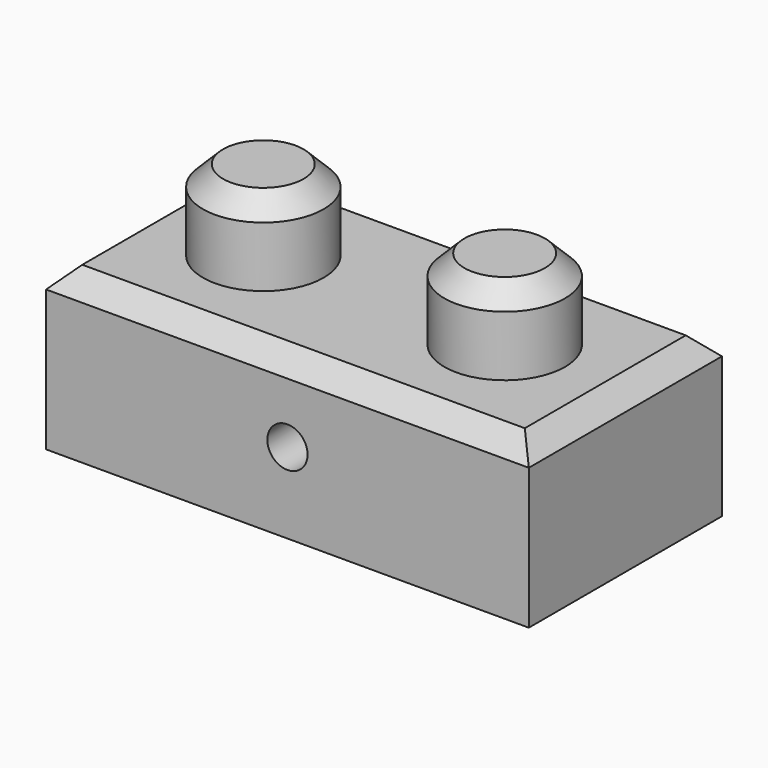
from build123d import *

# Parameters (mm, degrees)
F0_W     = 76.2
F0_H     = 38.1
F1_DEPTH = 25.4
F2_R     = 9.525
F3_DEPTH = 12.7
F4_SIZE2 = 3.175
F4_SIZE  = 3.175
F5_T     = 7.9375
F6_R     = 3.175
F7_DEPTH = 38.1


# Not quite as in the source:
# - a shell that OpenCascade refuses in one call is made with other operations: the cavity is built on its own and cut out


with BuildPart() as f1:
    # F0 (on Top) → F1 (new body)
    with BuildSketch(Plane.XY):
        with Locations((38.1, -19.05)):
            Rectangle(F0_W, F0_H)
    extrude(amount=F1_DEPTH)

    # F2 (on face) → F3 (join)
    with BuildSketch(Plane.XY.offset(25.4)):
        with Locations((19.05, -19.05)):
            Circle(F2_R)
        with Locations((57.15, -19.05)):
            Circle(F2_R)
    extrude(amount=F3_DEPTH)

    # F4
    f4_edges = [f1.edges().sort_by_distance(p)[0] for p in [
        (9.525, -19.05, 38.1),
        (47.625, -19.05, 38.1),
        (38.1, -38.1, 25.4),
        (76.2, -19.05, 25.4),
        (38.1, 0, 25.4),
        (0, -19.05, 25.4),
    ]]
    chamfer(f4_edges, length=F4_SIZE, length2=F4_SIZE2)

    # F5: shell of thickness 7.9375, made by hand


with BuildPart() as f5_core1:
    # F5_t2: copy of F1
    add(f1.part)

    # the walls: a layer under each face that stays
    f5_faces = [f5_core1.faces().sort_by_distance(p)[0] for p in [
        (38.1, 0, 11.1125),
        (76.2, -19.05, 11.1125),
        (38.1, -1.5875, 23.8125),
        (0, -19.05, 11.1125),
        (38.1, -38.1, 11.1125),
        (74.6125, -19.05, 23.8125),
        (38.1, -19.05, 25.4),
        (1.5875, -19.05, 23.8125),
        (38.1, -36.5125, 23.8125),
        (9.525, -19.05, 30.1625),
        (47.625, -19.05, 30.1625),
        (11.1125, -19.05, 36.5125),
        (49.2125, -19.05, 36.5125),
        (19.05, -19.05, 38.1),
        (57.15, -19.05, 38.1),
    ]]
    thicken(f5_faces, amount=-F5_T, mode=Mode.SUBTRACT)

    # F5_s3 → F5_t4 (revolve, cut)
    with BuildSketch(Plane.XZ.offset(19.05)):
        Polygon((28.654375, 25.479375), (28.575, 17.4625), (20.6375, 17.4625), (20.6375, 25.4), align=None)
    revolve(axis=Axis((19.05, -19.05, 25.4), (0, 0, 1)), mode=Mode.SUBTRACT)

    # F5_s5 → F5_t6 (revolve, cut)
    with BuildSketch(Plane.XZ.offset(19.05)):
        Polygon((66.754375, 25.479375), (66.675, 17.4625), (58.7375, 17.4625), (58.7375, 25.4), align=None)
    revolve(axis=Axis((57.15, -19.05, 25.4), (0, 0, 1)), mode=Mode.SUBTRACT)


with BuildPart() as f1_1:
    add(f1.part)

    # what is left inside the walls is the cavity
    f5_cavity = [f5_core1.part.solids().sort_by_distance(p)[0] for p in [
        (38.1, -22.754167, 0.079375),
    ]]
    add(f5_cavity, mode=Mode.SUBTRACT)

    # F6 (on face) → F7 (cut)
    with BuildSketch(Plane.XZ.offset(38.1)):
        with Locations((38.1, 12.7)):
            Circle(F6_R)
    extrude(amount=-F7_DEPTH, mode=Mode.SUBTRACT)


solid = f1_1.part
